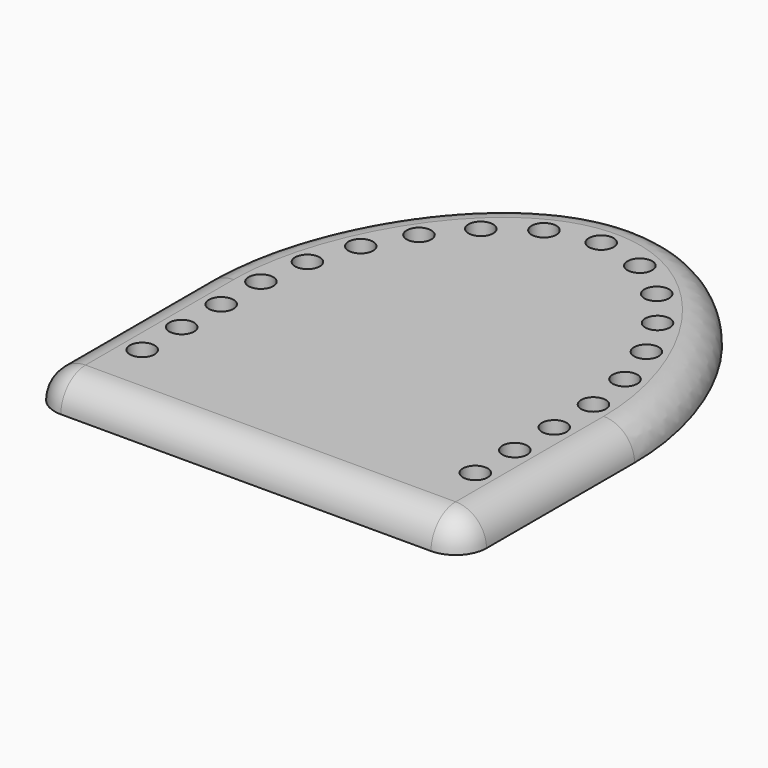
from build123d import *

# Parameters (mm, degrees)
F1_DEPTH = 5
F2_D     = 4
F3_R     = 4.9999


# Not quite as in the source:
# - a fillet or chamfer is up to 0.001 mm smaller than in the source, because OpenCascade refuses the exact size
# - ends of sketch curves that miss each other by under 0.0002 mm in the source are joined


with BuildPart() as f1:
    # F0 (on Top) → F1 (new body)
    with BuildSketch(Plane.XY):
        with BuildLine():
            Line((-35, 2.1762e-06), (-35, -35))
            Line((-35, -35), (-27, -35))
            Line((-27, -35), (-27, -22.2710574513))
            ThreePointArc((-27, -22.2710574513), (-32.9393385518, -11.8321585422), (-35, 2.1762e-06))
        make_face()
        with BuildLine():
            Line((-27, -22.2710574513), (-27, -35))
            Line((-27, -35), (0, -35))
            ThreePointArc((0, -35), (-14.9250291324, -31.658229663), (-27, -22.2710574513))
        make_face()
        with BuildLine():
            add(Edge.make_bspline(
                [(0, 45), (-20.1986748725, 45), (-35, 20.0504870868), (-35, 2.1762e-06)],
                knots=[0, 0, 0, 0, 57.0087695372, 57.0087695372, 57.0087695372, 57.0087695372], degree=3))
            ThreePointArc((-35, 2.1762e-06), (-28.4666369261, 20.3629708568), (-11.3056830814, 33.1237306181))
            add(Edge.make_bspline(
                [(0, 37), (-0.2833414452, 37.0069688983), (-1.1232932293, 37.0068386903), (-2.7957299856, 36.8864035146), (-4.9942322029, 36.3521195303), (-7.6997383876, 35.2871018647), (-9.7958540485, 34.148638444), (-11.0540635502, 33.3003360386), (-11.3056830814, 33.1237306181)],
                knots=[0, 0, 0, 0, 0.8506820357, 2.5185967411, 5.0181648841, 7.6012051941, 11.2266191262, 12.1476935207, 12.1476935207, 12.1476935207, 12.1476935207], degree=3))
            add(Edge.make_bspline(
                [(0, 37), (0.2833414452, 37.0069688983), (1.1232932293, 37.0068386903), (2.7957299856, 36.8864035146), (4.9942322029, 36.3521195303), (7.6997383876, 35.2871018647), (9.7958540485, 34.148638444), (11.0540635502, 33.3003360386), (11.3056830814, 33.1237306181)],
                knots=[0, 0, 0, 0, 0.8506820357, 2.5185967411, 5.0181648841, 7.6012051941, 11.2266191262, 12.1476935207, 12.1476935207, 12.1476935207, 12.1476935207], degree=3))
            ThreePointArc((11.3056830814, 33.1237306181), (28.4666375592, 20.3629699719), (35, 0))
            add(Edge.make_bspline(
                [(0, 45), (20.1986748725, 45), (35, 20.0504870868), (35, 0)],
                knots=[0, 0, 0, 0, 57.0087695372, 57.0087695372, 57.0087695372, 57.0087695372], degree=3))
        make_face()
        with BuildLine():
            ThreePointArc((-11.3056830814, 33.1237306181), (-28.4666369261, 20.3629708568), (-35, 2.1762e-06))
            ThreePointArc((-35, 2.1762e-06), (-32.9393385518, -11.8321585422), (-27, -22.2710574513))
            Line((-27, -22.2710574513), (-27, 2.1762e-06))
            add(Edge.make_bspline(
                [(-11.3056830814, 33.1237306181), (-12.4097508436, 32.3488132243), (-15.1414824386, 30.0752135158), (-18.8876274503, 25.5283101279), (-22.422035633, 19.604279738), (-25.0662594291, 13.1120426553), (-26.6478130576, 7.1844788974), (-27.0173066601, 2.7756083867), (-27.018694794, 0.6711028041), (-27, 2.1762e-06)],
                knots=[12.1476935207, 12.1476935207, 12.1476935207, 12.1476935207, 16.189226149, 22.7543847852, 29.7183326598, 36.8091409701, 43.7289829573, 48.0262708445, 50.0404462243, 50.0404462243, 50.0404462243, 50.0404462243], degree=3))
        make_face()
        with BuildLine():
            ThreePointArc((27, -22.2710574513), (14.9250291324, -31.658229663), (0, -35))
            Line((0, -35), (27, -35))
            Line((27, -35), (27, -22.2710574513))
        make_face()
        with BuildLine():
            ThreePointArc((-27, -22.2710574513), (-14.9250291324, -31.658229663), (0, -35))
            ThreePointArc((0, -35), (14.9250291324, -31.658229663), (27, -22.2710574513))
            Line((27, -22.2710574513), (27, 2.1762e-06))
            add(Edge.make_bspline(
                [(11.3056830814, 33.1237306181), (12.4097508436, 32.3488132243), (15.1414824386, 30.0752135158), (18.8876274503, 25.5283101279), (22.422035633, 19.604279738), (25.0662594291, 13.1120426553), (26.6478130576, 7.1844788974), (27.0173066601, 2.7756083867), (27.018694794, 0.6711028041), (27, 2.1762e-06)],
                knots=[12.1476935207, 12.1476935207, 12.1476935207, 12.1476935207, 16.189226149, 22.7543847852, 29.7183326598, 36.8091409701, 43.7289829573, 48.0262708445, 50.0404462243, 50.0404462243, 50.0404462243, 50.0404462243], degree=3))
            ThreePointArc((11.3056830814, 33.1237306181), (0, 35), (-11.3056830814, 33.1237306181))
            add(Edge.make_bspline(
                [(-11.3056830814, 33.1237306181), (-12.4097508436, 32.3488132243), (-15.1414824386, 30.0752135158), (-18.8876274503, 25.5283101279), (-22.422035633, 19.604279738), (-25.0662594291, 13.1120426553), (-26.6478130576, 7.1844788974), (-27.0173066601, 2.7756083867), (-27.018694794, 0.6711028041), (-27, 2.1762e-06)],
                knots=[12.1476935207, 12.1476935207, 12.1476935207, 12.1476935207, 16.189226149, 22.7543847852, 29.7183326598, 36.8091409701, 43.7289829573, 48.0262708445, 50.0404462243, 50.0404462243, 50.0404462243, 50.0404462243], degree=3))
            Line((-27, 2.1762e-06), (-27, -22.2710574513))
        make_face()
        with BuildLine():
            Line((27, -22.2710574513), (27, -35))
            Line((27, -35), (35, -35))
            Line((35, -35), (35, 0))
            ThreePointArc((35, 0), (32.939338184, -11.8321595662), (27, -22.2710574513))
        make_face()
        with BuildLine():
            Line((27, 2.1762e-06), (27, -22.2710574513))
            ThreePointArc((27, -22.2710574513), (32.939338184, -11.8321595662), (35, 0))
            ThreePointArc((35, 0), (28.4666375592, 20.3629699719), (11.3056830814, 33.1237306181))
            add(Edge.make_bspline(
                [(11.3056830814, 33.1237306181), (12.4097508436, 32.3488132243), (15.1414824386, 30.0752135158), (18.8876274503, 25.5283101279), (22.422035633, 19.604279738), (25.0662594291, 13.1120426553), (26.6478130576, 7.1844788974), (27.0173066601, 2.7756083867), (27.018694794, 0.6711028041), (27, 2.1762e-06)],
                knots=[12.1476935207, 12.1476935207, 12.1476935207, 12.1476935207, 16.189226149, 22.7543847852, 29.7183326598, 36.8091409701, 43.7289829573, 48.0262708445, 50.0404462243, 50.0404462243, 50.0404462243, 50.0404462243], degree=3))
        make_face()
        with BuildLine():
            add(Edge.make_bspline(
                [(0, 37), (-0.2833414452, 37.0069688983), (-1.1232932293, 37.0068386903), (-2.7957299856, 36.8864035146), (-4.9942322029, 36.3521195303), (-7.6997383876, 35.2871018647), (-9.7958540485, 34.148638444), (-11.0540635502, 33.3003360386), (-11.3056830814, 33.1237306181)],
                knots=[0, 0, 0, 0, 0.8506820357, 2.5185967411, 5.0181648841, 7.6012051941, 11.2266191262, 12.1476935207, 12.1476935207, 12.1476935207, 12.1476935207], degree=3))
            ThreePointArc((-11.3056830814, 33.1237306181), (0, 35), (11.3056830814, 33.1237306181))
            add(Edge.make_bspline(
                [(0, 37), (0.2833414452, 37.0069688983), (1.1232932293, 37.0068386903), (2.7957299856, 36.8864035146), (4.9942322029, 36.3521195303), (7.6997383876, 35.2871018647), (9.7958540485, 34.148638444), (11.0540635502, 33.3003360386), (11.3056830814, 33.1237306181)],
                knots=[0, 0, 0, 0, 0.8506820357, 2.5185967411, 5.0181648841, 7.6012051941, 11.2266191262, 12.1476935207, 12.1476935207, 12.1476935207, 12.1476935207], degree=3))
        make_face()
    extrude(amount=F1_DEPTH)

    # F2 (through all)
    with Locations(Plane(origin=(0, 0, 0), x_dir=(1, 0, 0), z_dir=(0, 0, -1))):
        with Locations((0, -37), (-7.7739062126, -35.111513252), (-14.2579257305, -30.4256311694), (-19.3371352018, -24.244884358), (-23.1543015859, -17.2142911543), (-25.7431047524, -9.6447404302), (-26.9552512695, -1.7371048277), (-27, 6.2627700182), (-27, 14.2627700182), (-27, 22.2627700182), (7.7739062126, -35.111513252), (14.2579257305, -30.4256311694), (19.3371352018, -24.244884358), (23.1543015859, -17.2142911543), (25.7431047524, -9.6447404302), (26.9552512695, -1.7371048277), (27, 6.2627700182), (27, 14.2627700182), (27, 22.2627700182)):
            Hole(F2_D / 2)

    # F3 (radius 5 in the source; OpenCascade refuses exactly that, so slightly less here)
    f3_edges = [f1.edges().sort_by_distance(p)[0] for p in [
        (-35, -35, 2.5),
        (35, -35, 2.5),
        (-35, -17.499999, 5),
        (0, -35, 5),
    ]]
    fillet(f3_edges, radius=F3_R)


solid = f1.part
